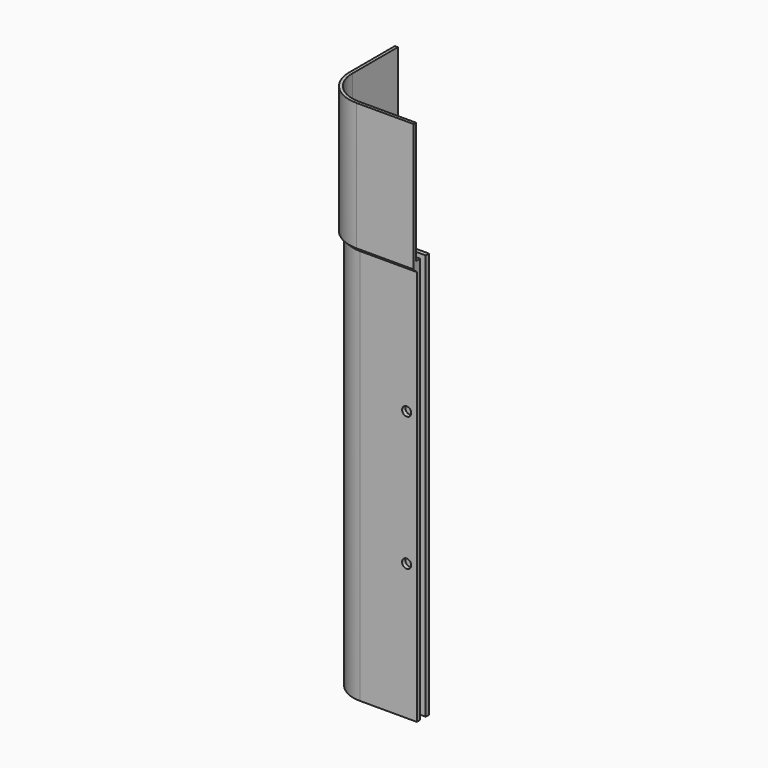
from build123d import *

# Parameters (mm, degrees)
F1_DEPTH       = 200
F2_T1_DEPTH    = 205.0938285461
F4_DEPTH       = 5
F5_SIZE        = 1.99999
F6_DEPTH       = 60
F7_R           = 2.25
F8_DEPTH       = 25
F8_DEPTH_BACK  = 25
F9_R           = 2.25
F10_DEPTH      = 25
F10_DEPTH_BACK = 25


# Not quite as in the source:
# - a fillet or chamfer that OpenCascade refuses, or shapes differently, is made with other operations: its cross-section is extruded or revolved along the edge and cut away or added
# - a fillet or chamfer is up to 0.001 mm smaller than in the source, because OpenCascade refuses the exact size


with BuildPart() as f1:
    # F0 (on Top) → F1 (new body)
    with BuildSketch(Plane.XY):
        with BuildLine():
            ThreePointArc((-13.2, 8.2159349274), (-15.426540085, 4.3732592746), (-16.2, 0))
            ThreePointArc((-16.2, 0), (-11.4551298552, -11.4551298552), (0, -16.2))
            ThreePointArc((0, -16.2), (4.3732592746, -15.426540085), (8.2159349274, -13.2))
            Line((8.2159349274, -13.2), (0, -13.2))
            ThreePointArc((0, -13.2), (-9.3338095117, -9.3338095117), (-13.2, 0))
            Line((-13.2, 0), (-13.2, 8.2159349274))
        make_face()
        with BuildLine():
            Line((-16.2, 12), (-16.2, 0))
            ThreePointArc((-16.2, 0), (-15.426540085, 4.3732592746), (-13.2, 8.2159349274))
            Line((-13.2, 8.2159349274), (-13.2, 12))
            Line((-13.2, 12), (-8.7, 16.5))
            Line((-8.7, 16.5), (-8.7, 28))
            Line((-8.7, 28), (-10.7, 28))
            Line((-10.7, 28), (-10.7, 18))
            Line((-10.7, 18), (-14.2, 18))
            Line((-14.2, 18), (-14.2, 28))
            Line((-14.2, 28), (-16.2, 28))
            Line((-16.2, 28), (-16.2, 12))
        make_face()
        with BuildLine():
            ThreePointArc((8.2159349274, -13.2), (4.3732592746, -15.426540085), (0, -16.2))
            Line((0, -16.2), (12, -16.2))
            Line((12, -16.2), (28, -16.2))
            Line((28, -16.2), (28, -14.2))
            Line((28, -14.2), (18, -14.2))
            Line((18, -14.2), (18, -10.7))
            Line((18, -10.7), (28, -10.7))
            Line((28, -10.7), (28, -8.7))
            Line((28, -8.7), (16.5, -8.7))
            Line((16.5, -8.7), (12, -13.2))
            Line((12, -13.2), (8.2159349274, -13.2))
        make_face()
        with BuildLine():
            ThreePointArc((-3.4164113954, 12.750220907), (-8.8111411033, 11.568257177), (-13.2, 8.2159349274))
            Line((-13.2, 8.2159349274), (-13.2, 0))
            ThreePointArc((-13.2, 0), (-10.4722640918, 8.0356508629), (-3.4164113954, 12.750220907))
        make_face()
        with BuildLine():
            Line((0, -13.2), (8.2159349274, -13.2))
            ThreePointArc((8.2159349274, -13.2), (11.568257177, -8.8111411033), (12.750220907, -3.4164113954))
            ThreePointArc((12.750220907, -3.4164113954), (8.0356508629, -10.4722640918), (0, -13.2))
        make_face()
    extrude(amount=F1_DEPTH)

    # F2: chamfer of 1 on 2 edges, made by hand

    # F2_s2 → F2_t1 (cut)
    with BuildSketch(Plane.XY.offset(-2.546914273)):
        with BuildLine():
            Line((-4.3644750665, 12.4155520043), (-4.4351757111, 12.7519059003))
            Line((-4.4351757111, 12.7519059003), (-4.436708561, 12.7718470731))
            ThreePointArc((-4.436708561, 12.7718470731), (-3.9261784824, 12.7613736088), (-3.4163591233, 12.7702208387))
            Line((-3.4163591233, 12.7702208387), (-3.4112350145, 12.7309023905))
            ThreePointArc((-3.4112350145, 12.7309023905), (-3.893221277, 12.5918715086), (-4.3578497587, 12.3966812519))
            Line((-4.3578497587, 12.3966812519), (-4.3644750665, 12.4155520043))
        make_face()
        with BuildLine():
            Line((12.7519059003, -4.4351757111), (12.4155520043, -4.3644750665))
            Line((12.4155520043, -4.3644750665), (12.3966812519, -4.3578497587))
            ThreePointArc((12.3966812519, -4.3578497587), (12.5918715086, -3.893221277), (12.7309023905, -3.4112350145))
            Line((12.7309023905, -3.4112350145), (12.7702208387, -3.4163591233))
            ThreePointArc((12.7702208387, -3.4163591233), (12.7613736088, -3.9261784824), (12.7718470731, -4.436708561))
            Line((12.7718470731, -4.436708561), (12.7519059003, -4.4351757111))
        make_face()
    extrude(amount=F2_T1_DEPTH, mode=Mode.SUBTRACT)

    # F3 (on face) → F4 (join)
    with BuildSketch(Plane.XY.offset(200)):
        with BuildLine():
            Line((28, -16.7), (28, -16.2))
            Line((28, -16.2), (0, -16.2))
            ThreePointArc((0, -16.2), (-11.4551298552, -11.4551298552), (-16.2, 0))
            Line((-16.2, 0), (-16.2, 28))
            Line((-16.2, 28), (-16.7, 28))
            Line((-16.7, 28), (-16.7, 0))
            ThreePointArc((-16.7, 0), (-11.8086832458, -11.8086832458), (0, -16.7))
            Line((0, -16.7), (28, -16.7))
        make_face()
        with BuildLine():
            Line((28, -18.2), (28, -16.7))
            Line((28, -16.7), (0, -16.7))
            ThreePointArc((0, -16.7), (-11.8086832458, -11.8086832458), (-16.7, 0))
            Line((-16.7, 0), (-16.7, 28))
            Line((-16.7, 28), (-18.2, 28))
            Line((-18.2, 28), (-18.2, 0))
            ThreePointArc((-18.2, 0), (-12.8693434176, -12.8693434176), (0, -18.2))
            Line((0, -18.2), (28, -18.2))
        make_face()
    extrude(amount=-F4_DEPTH)

    # F5 (size 2 in the source; OpenCascade refuses exactly that, so slightly less here)
    f5_edges = [f1.edges().sort_by_distance(p)[0] for p in [
        (-18.2, 14, 195),
        (-12.869343, -12.869343, 195),
        (14, -18.2, 195),
    ]]
    chamfer(f5_edges, length=F5_SIZE)

    # F3 (on face) → F6 (join)
    with BuildSketch(Plane.XY.offset(200)):
        with BuildLine():
            Line((28, -18.2), (28, -16.7))
            Line((28, -16.7), (0, -16.7))
            ThreePointArc((0, -16.7), (-11.8086832458, -11.8086832458), (-16.7, 0))
            Line((-16.7, 0), (-16.7, 28))
            Line((-16.7, 28), (-18.2, 28))
            Line((-18.2, 28), (-18.2, 0))
            ThreePointArc((-18.2, 0), (-12.8693434176, -12.8693434176), (0, -18.2))
            Line((0, -18.2), (28, -18.2))
        make_face()
    extrude(amount=F6_DEPTH)

    # F7 (on face) → F8 (cut, two sides)
    with BuildSketch(Plane(origin=(0, -14.2, 0), x_dir=(-1, 0, 0), z_dir=(0, 1, 0))) as f8_sk:
        with Locations((-23, 133)):
            Circle(F7_R)
        with Locations((-23, 67)):
            Circle(F7_R)
    extrude(amount=-F8_DEPTH, mode=Mode.SUBTRACT)
    extrude(f8_sk.sketch, amount=F8_DEPTH_BACK, mode=Mode.SUBTRACT)

    # F9 (on face) → F10 (cut, two sides)
    with BuildSketch(Plane.YZ.offset(-14.2)) as f10_sk:
        with Locations((23, 133)):
            Circle(F9_R)
        with Locations((23, 67)):
            Circle(F9_R)
    extrude(amount=-F10_DEPTH, mode=Mode.SUBTRACT)
    extrude(f10_sk.sketch, amount=F10_DEPTH_BACK, mode=Mode.SUBTRACT)


solid = f1.part
